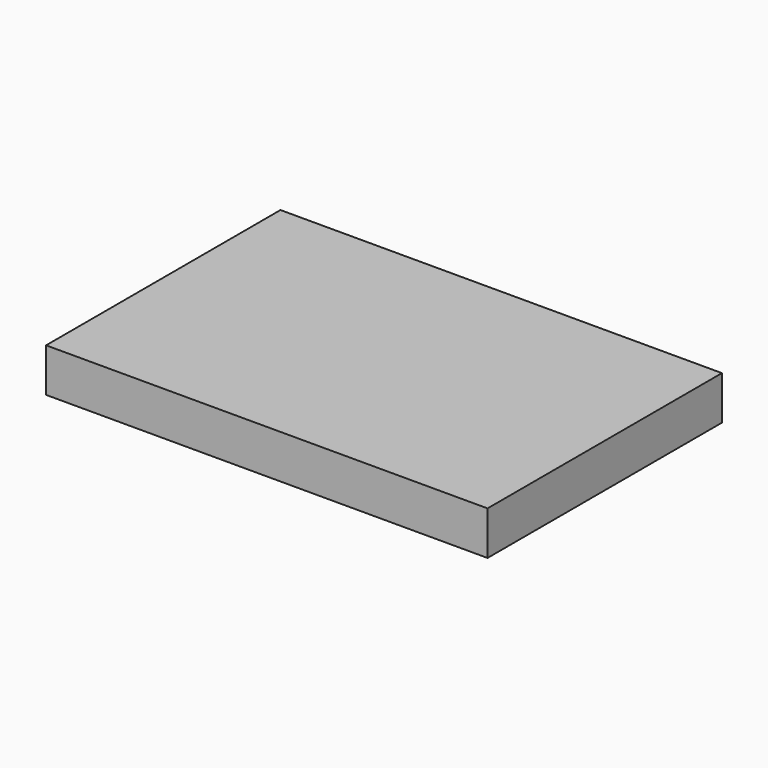
from build123d import *

# Parameters (mm, degrees)
F0_W     = 64.2119571567
F0_H     = 42.6151417196
F1_DEPTH = 6.35


# Not quite as in the source:
# - the program builds the solid bodies; features that only make, move or delete a surface that nothing else refers to are left out


with BuildPart() as f1:
    # F0 (on Top) → F1 (new body)
    with BuildSketch(Plane.XY):
        Rectangle(F0_W, F0_H)
    extrude(amount=F1_DEPTH)


solid = f1.part
